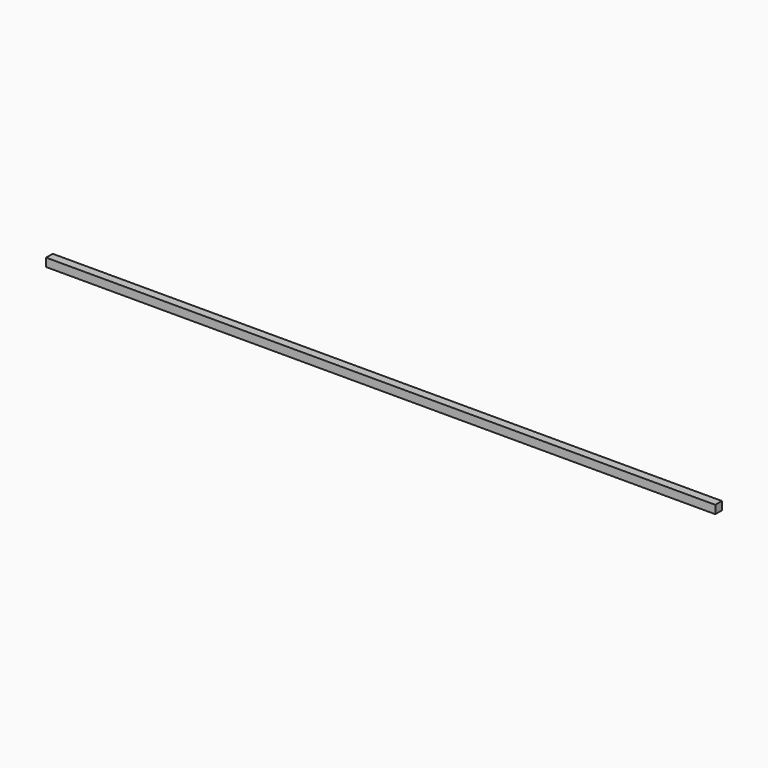
from build123d import *

# Parameters (mm, degrees)
F0_W     = 256.032
F0_H     = 3.175
F1_DEPTH = 3.175


# Not quite as in the source:
# - a length typed as a fraction of an inch, garbled in the dataset ("3 / 203.2 mm" for 3/8 in), is restored


with BuildPart() as f1:
    # F0 (on Front) → F1 (new body)
    with BuildSketch(Plane.XZ):
        with Locations((22.9623306289, -8.6084658129)):
            Rectangle(F0_W, F0_H)
    extrude(amount=F1_DEPTH)


solid = f1.part
